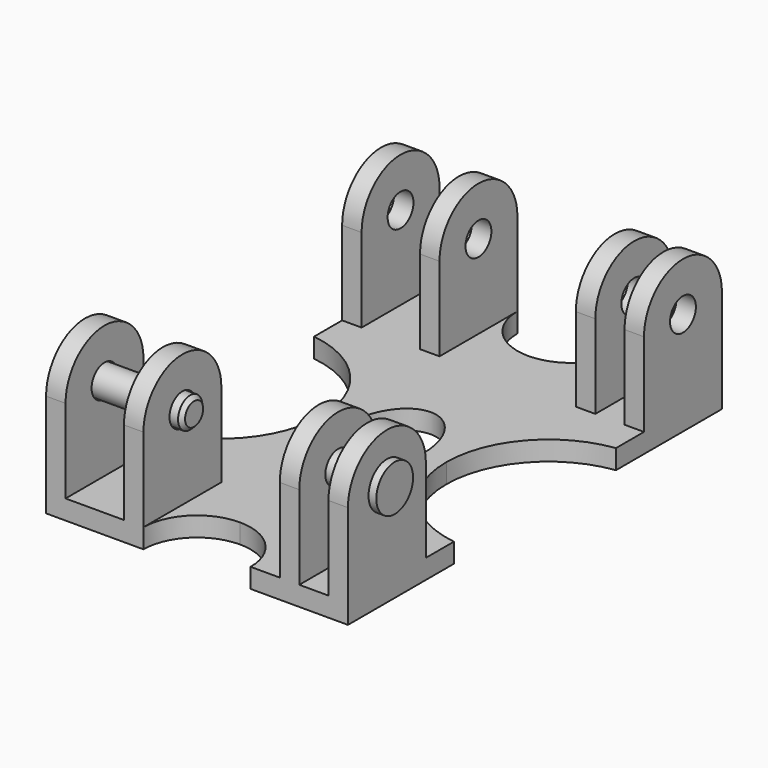
from build123d import *

# Parameters (mm, degrees)
F3_DEPTH   = 5
F6_R       = 4.15
F7_DEPTH   = 5
F9_R       = 4.15
F10_DEPTH  = 5
F13_R      = 4.15
F14_DEPTH  = 5
F15_R      = 4.15
F16_DEPTH  = 5
F17_R      = 3.9
F18_DEPTH  = 20.5
F19_R      = 5.9
F20_DEPTH  = 2
F21_R      = 3.9
F22_DEPTH  = 28
F23_R      = 5.9
F24_DEPTH  = 2
F25_SIZE   = 1
F25_2_SIZE = 1


# Not quite as in the source:
# - a pattern or mirror of a feature is missing from the dataset's text; its kind, count and spacing are read off the source's solid


with BuildPart() as f3:
    # F2 (on Top) → F3 (new body)
    with BuildSketch(Plane.XY):
        with BuildLine():
            ThreePointArc((38.75, -26), (22.4904434906, -17.2739869457), (16, 0))
            ThreePointArc((16, 0), (22.4904434906, 17.2739869457), (38.75, 26))
            Line((38.75, 26), (38.75, 60))
            Line((38.75, 60), (13.75, 60))
            ThreePointArc((13.75, 60), (9.7227182413, 50.2772817587), (0, 46.25))
            ThreePointArc((0, 46.25), (-9.7227182413, 50.2772817587), (-13.75, 60))
            Line((-13.75, 60), (-38.75, 60))
            Line((-38.75, 60), (-38.75, 26))
            ThreePointArc((-38.75, 26), (-22.4904434906, 17.2739869457), (-16, 0))
            ThreePointArc((-16, 0), (-22.4904434906, -17.2739869457), (-38.75, -26))
            Line((-38.75, -26), (-38.75, -60))
            Line((-38.75, -60), (-13.75, -60))
            ThreePointArc((-13.75, -60), (-9.7227182413, -50.2772817587), (0, -46.25))
            ThreePointArc((0, -46.25), (9.7227182413, -50.2772817587), (13.75, -60))
            Line((13.75, -60), (38.75, -60))
            Line((38.75, -60), (38.75, -26))
        make_face()
        with BuildLine():
            add(Edge.make_bspline(
                [(0, 15), (-17.3205080757, 15), (-8.6602540378, -7.5), (0, -30), (8.6602540378, -7.5), (17.3205080757, 15), (0, 15)],
                knots=[0, 0, 0, 2.0943951024, 2.0943951024, 4.1887902048, 4.1887902048, 6.2831853072, 6.2831853072, 6.2831853072], degree=2, weights=[1, 0.5, 1, 0.5, 1, 0.5, 1]))
        make_face(mode=Mode.SUBTRACT)
    extrude(amount=F3_DEPTH)

    # F6 (on offset) → F7 (join)
    with BuildSketch(Plane.YZ.offset(38.75)):
        with BuildLine():
            Line((-60, 5), (-35, 5))
            Line((-35, 5), (-35, 26.5))
            ThreePointArc((-35, 26.5), (-47.5, 39), (-60, 26.5))
            Line((-60, 26.5), (-60, 5))
        make_face()
        with Locations((-47.5, 26.5)):
            Circle(F6_R, mode=Mode.SUBTRACT)
    f7 = extrude(amount=-F7_DEPTH)

    # F7_copies: F7 across plane
    add(f7.mirror(Plane.ZX))

    # F9 (on offset) → F10 (join)
    with BuildSketch(Plane.YZ.offset(26.25)):
        with BuildLine():
            Line((-60, 5), (-35, 5))
            Line((-35, 5), (-35, 26.5))
            ThreePointArc((-35, 26.5), (-47.5, 39), (-60, 26.5))
            Line((-60, 26.5), (-60, 5))
        make_face()
        with Locations((-47.5, 26.5)):
            Circle(F9_R, mode=Mode.SUBTRACT)
    f10 = extrude(amount=-F10_DEPTH)

    # F10_copies: F10 across plane
    add(f10.mirror(Plane.ZX))

    # F13 (on offset) → F14 (join)
    with BuildSketch(Plane(origin=(-38.75, 0, 0), x_dir=(0, -1, 0), z_dir=(-1, 0, 0))):
        with BuildLine():
            Line((35, 26.5), (35, 5))
            Line((35, 5), (60, 5))
            Line((60, 5), (60, 26.5))
            ThreePointArc((60, 26.5), (47.5, 39), (35, 26.5))
        make_face()
        with Locations((47.5, 26.5)):
            Circle(F13_R, mode=Mode.SUBTRACT)
    f14 = extrude(amount=-F14_DEPTH)

    # F14_copies: F14 across plane
    add(f14.mirror(Plane.ZX))

    # F15 (on offset) → F16 (join)
    with BuildSketch(Plane(origin=(-18.75, 0, 0), x_dir=(0, -1, 0), z_dir=(-1, 0, 0))):
        with BuildLine():
            Line((35, 26.5), (35, 5))
            Line((35, 5), (60, 5))
            Line((60, 5), (60, 26.5))
            ThreePointArc((60, 26.5), (47.5, 39), (35, 26.5))
        make_face()
        with Locations((47.5, 26.5)):
            Circle(F15_R, mode=Mode.SUBTRACT)
    f16 = extrude(amount=-F16_DEPTH)

    # F16_copies: F16 across plane
    add(f16.mirror(Plane.ZX))


with BuildPart() as f18:
    # F17 (on face) → F18 (new body, through all)
    with BuildSketch(Plane.YZ.offset(38.75)):
        with Locations((-47.5, 26.5)):
            Circle(F17_R)
    extrude(amount=-F18_DEPTH)

    # F19 (on face) → F20 (join)
    with BuildSketch(Plane.YZ.offset(38.75)):
        with Locations((-47.5, 26.5)):
            Circle(F19_R)
    extrude(amount=F20_DEPTH)

    # F25
    f25_edges = [f18.edges().sort_by_distance(p)[0] for p in [
        (18.25, -51.4, 26.5),
        (38.75, -51.4, 26.5),
    ]]
    chamfer(f25_edges, length=F25_SIZE)


with BuildPart() as f22:
    # F21 (on face) → F22 (new body, through all)
    with BuildSketch(Plane(origin=(-38.75, 0, 0), x_dir=(0, -1, 0), z_dir=(-1, 0, 0))):
        with Locations((47.5, 26.5)):
            Circle(F21_R)
    extrude(amount=-F22_DEPTH)

    # F23 (on face) → F24 (join)
    with BuildSketch(Plane(origin=(-38.75, 0, 0), x_dir=(0, -1, 0), z_dir=(-1, 0, 0))):
        with Locations((47.5, 26.5)):
            Circle(F23_R)
    extrude(amount=F24_DEPTH)

    # F25#2
    f25_2_edges = [f22.edges().sort_by_distance(p)[0] for p in [
        (-38.75, -43.6, 26.5),
        (-10.75, -43.6, 26.5),
    ]]
    chamfer(f25_2_edges, length=F25_2_SIZE)


solid = Compound([f3.part, f18.part, f22.part])
